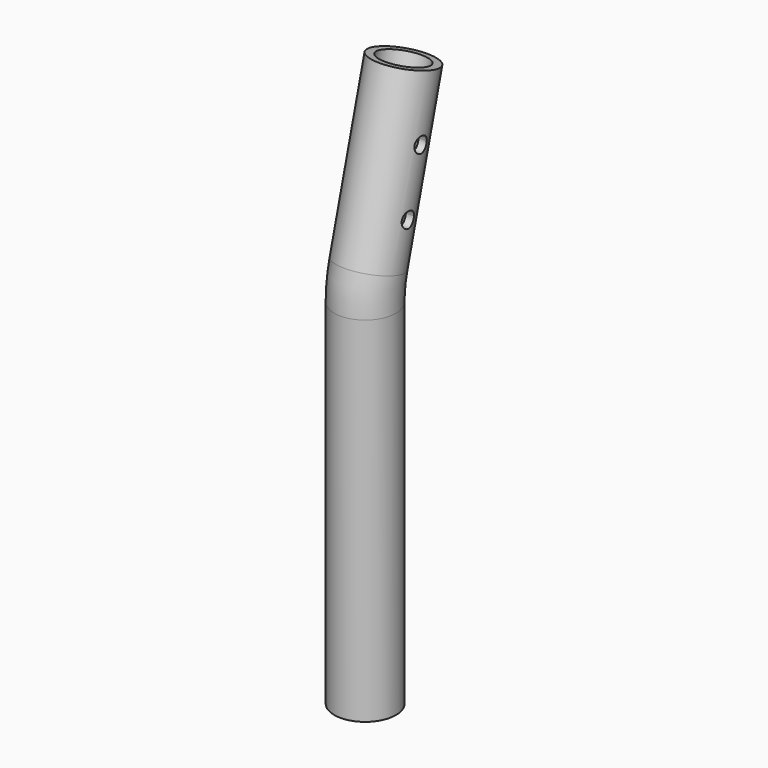
from build123d import *

# Parameters (mm, degrees)
F0_R     = 12.7
F0_R_2   = 9.525
F3_DEPTH = 25.4


with BuildPart() as f2:
    # F2: sweep along a path in F1
    with BuildLine(Plane.YZ) as f2_path:
        Line((0, 0), (0, 145.7120531226))
        ThreePointArc((0, 145.7120531226), (0.4346010422, 152.3427836873), (1.7309680245, 158.8600606138))
        Line((1.7309680245, 158.8600606138), (19.7220112368, 226.0035479632))
    # F0 (on Top) → F2 (sweep)
    with BuildSketch(Plane.XY):
        Circle(F0_R)
        Circle(F0_R_2, mode=Mode.SUBTRACT)
    sweep(path=f2_path.line)

    # F1 (on Right) → F3 (cut, symmetric)
    with BuildSketch(Plane.YZ):
        with BuildLine():
            ThreePointArc((13.9697579594, 204.535846474), (10.0811929927, 202.2907824437), (12.326257023, 198.402217477))
            Line((12.326257023, 198.402217477), (13.9697579594, 204.535846474))
        make_face()
        with BuildLine():
            Line((13.9697579594, 204.535846474), (12.326257023, 198.402217477))
            ThreePointArc((12.326257023, 198.402217477), (15.0808250283, 198.9501351201), (16.3230074912, 201.4690319755))
            ThreePointArc((16.3230074912, 201.4690319755), (15.6669043466, 203.4018495126), (13.9697579594, 204.535846474))
        make_face()
        with BuildLine():
            Line((7.3957542138, 180.0013304862), (5.7522532774, 173.8677014893))
            ThreePointArc((5.7522532774, 173.8677014893), (8.5068212827, 174.4156191323), (9.7490037456, 176.9345159877))
            ThreePointArc((9.7490037456, 176.9345159877), (9.092900601, 178.8673335248), (7.3957542138, 180.0013304862))
        make_face()
        with BuildLine():
            ThreePointArc((7.3957542138, 180.0013304862), (3.5071892471, 177.7562664559), (5.7522532774, 173.8677014893))
            Line((5.7522532774, 173.8677014893), (7.3957542138, 180.0013304862))
        make_face()
    extrude(amount=F3_DEPTH, both=True, mode=Mode.SUBTRACT)


solid = f2.part
